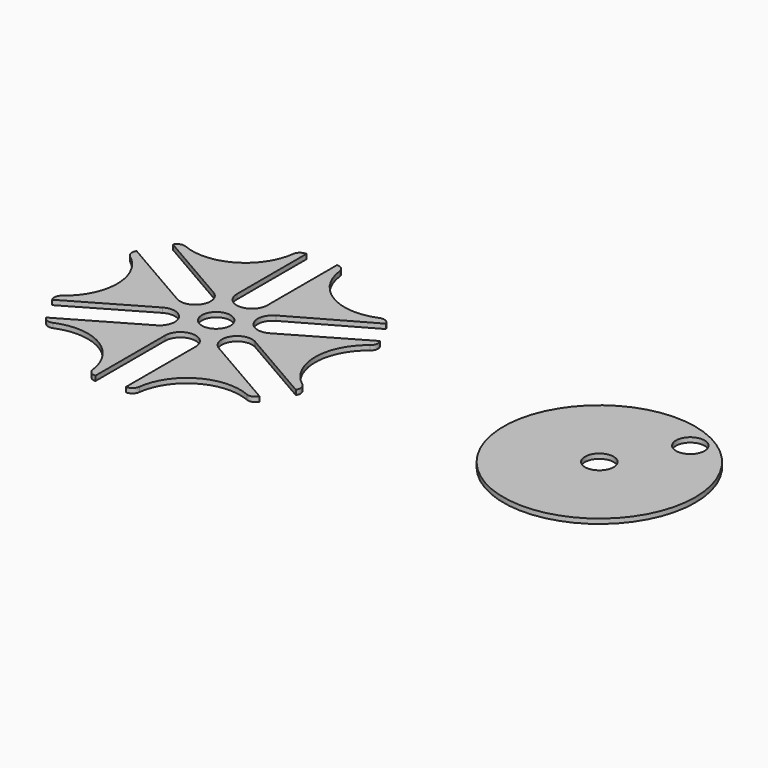
from build123d import *

# Parameters (mm, degrees)
F0_R     = 9.525
F1_DEPTH = 3.175
F2_R     = 5.08
F0_R_2   = 63.9582216699
F0_R_3   = 33.02
F3_DEPTH = 3.175


# Not quite as in the source:
# - a length typed as a fraction of an inch, garbled in the dataset ("3 / 203.2 mm" for 3/8 in), is restored
# - a feature names something its author has since deleted; it is built from what else it names


with BuildPart() as f1:
    # F0 (on Top) → F1 (new body)
    with BuildSketch(Plane.XY):
        with BuildLine():
            ThreePointArc((-17.78, -30.7958633586), (-35.5599563921, -0.0556901267), (-17.8763707949, 30.7400222382))
            Line((-17.8763707949, 30.7400222382), (-20.4296415334, 35.1306001794))
            Line((-20.4296415334, 35.1306001794), (-70.6329627114, 6.1469720917))
            ThreePointArc((-70.6329627114, 6.1469720917), (-84.5232381264, 9.8860746707), (-80.7525608015, 23.7678120156))
            ThreePointArc((-80.7525608015, 23.7678120156), (-80.7108842522, 23.7914906594), (-80.6690964546, 23.8149724163))
            Line((-80.6690964546, 23.8149724163), (-30.2104125797, 52.3259695061))
            Line((-30.2104125797, 52.3259695061), (-33.0188105519, 57.1902574851))
            ThreePointArc((-33.0188105519, 57.1902574851), (-68.5788105527, 57.1902574837), (-86.3588105535, 87.9861208428))
            Line((-86.3588105535, 87.9861208428), (-91.4394053355, 87.9861208428))
            Line((-91.4394053355, 87.9861208428), (-91.4394053355, 29.8429398183))
            ThreePointArc((-91.4394053355, 29.8429398183), (-101.6004354264, 19.6829398705), (-111.7594051266, 29.845))
            Line((-111.7594051266, 29.845), (-111.7594051266, 87.9881810245))
            Line((-111.7594051266, 87.9881810245), (-116.84, 87.9881810245))
            ThreePointArc((-116.84, 87.9881810245), (-134.62, 57.1923176659), (-170.18, 57.1923176659))
            Line((-170.18, 57.1923176659), (-172.7201599914, 52.7926315014))
            Line((-172.7201599914, 52.7926315014), (-122.4365198362, 23.7613583219))
            ThreePointArc((-122.4365198362, 23.7613583219), (-118.627620527, 9.8774561073), (-132.5265281759, 6.1236818976))
            Line((-132.5265281759, 6.1236818976), (-182.88, 35.1952724098))
            Line((-182.88, 35.1952724098), (-185.42, 30.7958633586))
            ThreePointArc((-185.42, 30.7958633586), (-167.64, 0), (-185.42, -30.7958633586))
            Line((-185.42, -30.7958633586), (-182.8800000009, -35.1952724082))
            Line((-182.8800000009, -35.1952724082), (-132.5258080212, -6.1245428478))
            ThreePointArc((-132.5258080212, -6.1245428478), (-118.6470606402, -9.8436248763), (-122.3661426686, -23.7223722573))
            Line((-122.3661426686, -23.7223722573), (-172.7194471607, -52.7938661604))
            Line((-172.7194471607, -52.7938661604), (-170.18, -57.1923176659))
            ThreePointArc((-170.18, -57.1923176659), (-134.62, -57.1923176659), (-116.84, -87.9881810245))
            Line((-116.84, -87.9881810245), (-111.76, -87.9881810245))
            Line((-111.76, -87.9881810245), (-111.76, -29.845))
            ThreePointArc((-111.76, -29.845), (-101.6, -19.685), (-91.44, -29.845))
            Line((-91.44, -29.845), (-91.4399999997, -87.9881810245))
            Line((-91.4399999997, -87.9881810245), (-86.36, -87.9881810245))
            ThreePointArc((-86.36, -87.9881810245), (-68.58, -57.1923176659), (-33.02, -57.1923176659))
            Line((-33.02, -57.1923176659), (-30.4777274407, -52.7889724266))
            Line((-30.4777274407, -52.7889724266), (-80.5680413022, -23.8693162349))
            ThreePointArc((-80.5680413022, -23.8693162349), (-84.7865541797, -10.2717986383), (-71.2681836795, -5.8061525812))
            ThreePointArc((-71.2681836795, -5.8061525812), (-70.6734718241, -6.1236818976), (-70.1011274419, -6.4799528141))
            Line((-70.1011274419, -6.4799528141), (-20.3311837367, -35.2146432099))
            Line((-20.3311837367, -35.2146432099), (-17.78, -30.7958633586))
        make_face()
        with Locations((-101.6, 0)):
            Circle(F0_R, mode=Mode.SUBTRACT)
    extrude(amount=F1_DEPTH)

    # F2
    f2_edges = [f1.edges().sort_by_distance(p)[0] for p in [
        (-17.876371, 30.740022, 1.5875),
        (-17.78, -30.795863, 1.5875),
        (-33.02, -57.192318, 1.5875),
        (-86.36, -87.988181, 1.5875),
        (-116.84, -87.988181, 1.5875),
        (-170.18, -57.192318, 1.5875),
        (-185.42, -30.795863, 1.5875),
        (-185.42, 30.795863, 1.5875),
        (-116.84, 87.988181, 1.5875),
        (-86.358811, 87.986121, 1.5875),
        (-33.018811, 57.190257, 1.5875),
        (-170.18, 57.192318, 1.5875),
    ]]
    fillet(f2_edges, radius=F2_R)


with BuildPart() as f3:
    # F0 (on Top) → F3 (new body)
    with BuildSketch(Plane.XY):
        with Locations((153.9702564478, 0)):
            Circle(F0_R_2)
        with Locations((153.9702564478, 0)):
            Circle(F0_R_3, mode=Mode.SUBTRACT)
        with Locations((179.5079290119, 43.9143174831)):
            Circle(F0_R, mode=Mode.SUBTRACT)
        with Locations((153.9702564478, 0)):
            Circle(F0_R_3)
        with Locations((153.9702564478, 0)):
            Circle(F0_R, mode=Mode.SUBTRACT)
    extrude(amount=F3_DEPTH)


solid = Compound([f1.part, f3.part])
